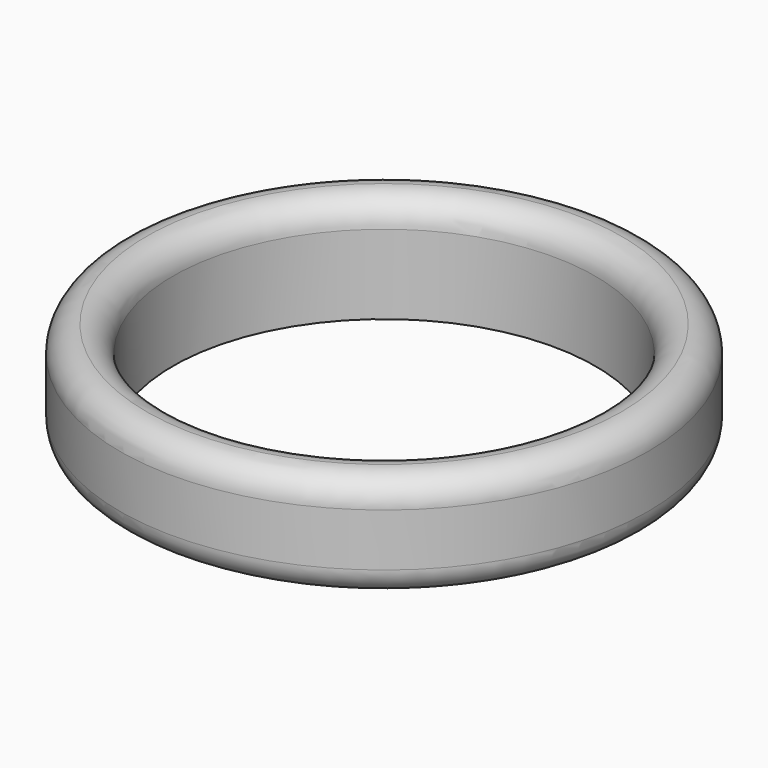
from build123d import *

# Parameters (mm, degrees)
F0_R     = 12.5
F0_R_2   = 10
F1_DEPTH = 5
F2_R     = 1.24999


# Not quite as in the source:
# - a fillet or chamfer is up to 0.001 mm smaller than in the source, because OpenCascade refuses the exact size


with BuildPart() as f1:
    # F0 (on Top) → F1 (new body)
    with BuildSketch(Plane.XY):
        Circle(F0_R)
        Circle(F0_R_2, mode=Mode.SUBTRACT)
    extrude(amount=F1_DEPTH)

    # F2 (radius 1.25 in the source; OpenCascade refuses exactly that, so slightly less here)
    f2_edges = [f1.edges().sort_by_distance(p)[0] for p in [
        (-10, 0, 5),
        (-12.5, 0, 5),
        (-12.5, 0, 0),
        (12.5, 0, 2.5),
    ]]
    fillet(f2_edges, radius=F2_R)


solid = f1.part
